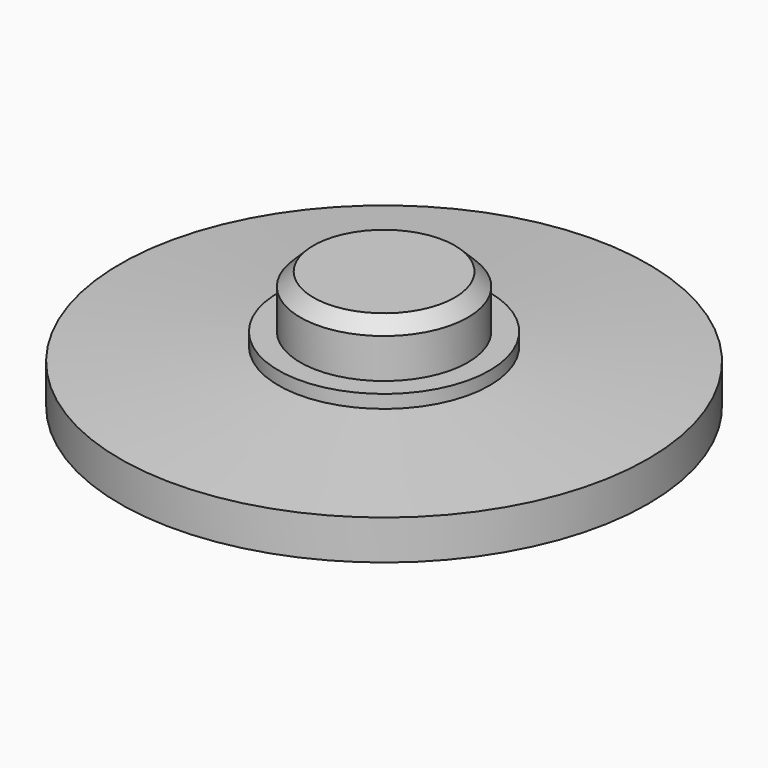
from build123d import *

# Parameters (mm, degrees)
F0_R     = 10
F1_DEPTH = 2
F2_R     = 4
F3_DEPTH = 0.5
F4_R     = 3.175
F5_DEPTH = 2
F6_R     = 9
F6_R_2   = 8
F6_R_3   = 7
F6_R_4   = 6
F6_R_5   = 5
F6_R_6   = 4
F7_DEPTH = 0.5
F8_SIZE2 = 0.49999
F8_SIZE  = 5.99999
F9_SIZE  = 0.5


# Not quite as in the source:
# - a fillet or chamfer is up to 0.001 mm smaller than in the source, because OpenCascade refuses the exact size


with BuildPart() as f1:
    # F0 (on Top) → F1 (new body)
    with BuildSketch(Plane.XY):
        Circle(F0_R)
    extrude(amount=F1_DEPTH)

    # F2 (on face) → F3 (join)
    with BuildSketch(Plane.XY.offset(2)):
        Circle(F2_R)
    extrude(amount=F3_DEPTH)

    # F4 (on face) → F5 (join)
    with BuildSketch(Plane.XY.offset(2.5)):
        Circle(F4_R)
    extrude(amount=F5_DEPTH)

    # F6 (on face) → F7 (cut)
    with BuildSketch(Plane(origin=(0, 0, 0), x_dir=(1, 0, 0), z_dir=(0, 0, -1))):
        Circle(F6_R)
        Circle(F6_R_2, mode=Mode.SUBTRACT)
        Circle(F6_R_3)
        Circle(F6_R_4, mode=Mode.SUBTRACT)
        Circle(F6_R_5)
        Circle(F6_R_6, mode=Mode.SUBTRACT)
    extrude(amount=-F7_DEPTH, mode=Mode.SUBTRACT)

    # F8 (size 6 and 0.5 in the source; OpenCascade refuses exactly that, so slightly less here)
    f8_edges = [f1.edges().sort_by_distance(p)[0] for p in [
        (-10, 0, 2),
    ]]
    f8_side = f1.faces().sort_by_distance((-9.717157, 0, 2))[0]
    chamfer(f8_edges, length=F8_SIZE, length2=F8_SIZE2, reference=f8_side)

    # F9
    f9_edges = [f1.edges().sort_by_distance(p)[0] for p in [
        (-3.175, 0, 4.5),
    ]]
    chamfer(f9_edges, length=F9_SIZE)


solid = f1.part
